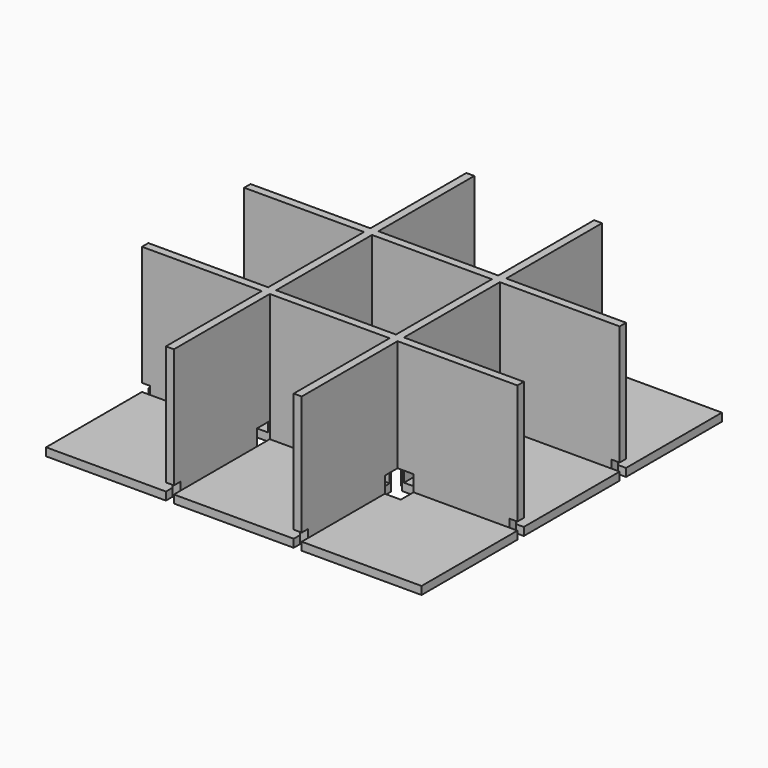
from build123d import *

# Parameters (mm, degrees)
F0_W     = 1
F0_H     = 15
F0_W_2   = 15
F0_H_2   = 1
F1_DEPTH = 1
F2_DEPTH = 16
F3_W     = 2
F3_H     = 3
F3_W_2   = 3
F3_H_2   = 2
F4_DEPTH = 3
F5_W     = 1
F5_H     = 1
F6_DEPTH = 25
F7_DEPTH = 15
F9_DEPTH = 1


with BuildPart() as f1:
    # F0 (on Top) → F1 (new body)
    with BuildSketch(Plane.XY):
        with Locations((8, 0)):
            Rectangle(F0_W, F0_H)
        with Locations((-16, -8)):
            Rectangle(F0_W_2, F0_H_2)
        with Locations((-16, 0)):
            Rectangle(F0_W_2, F0_H)
        with Locations((8, -16)):
            Rectangle(F0_W, F0_H)
        with Locations((0, -16)):
            Rectangle(F0_W_2, F0_H)
        with Locations((-8, -16)):
            Rectangle(F0_W, F0_H)
        with Locations((16, -16)):
            Rectangle(F0_W_2, F0_H)
        with Locations((-16, -16)):
            Rectangle(F0_W_2, F0_H)
        with Locations((16, 0)):
            Rectangle(F0_W_2, F0_H)
        with Locations((16, -8)):
            Rectangle(F0_W_2, F0_H_2)
        with Locations((0, -8)):
            Rectangle(F0_W_2, F0_H_2)
        with Locations((-8, 0)):
            Rectangle(F0_W, F0_H)
        Rectangle(F0_W_2, F0_H)
        with Locations((8, -8)):
            Rectangle(F0_W, F0_H_2)
        with Locations((-8, -8)):
            Rectangle(F0_W, F0_H_2)
        with Locations((-8, 8)):
            Rectangle(F0_W, F0_H_2)
        with Locations((-16, 8)):
            Rectangle(F0_W_2, F0_H_2)
        with Locations((8, 16)):
            Rectangle(F0_W, F0_H)
        with Locations((0, 16)):
            Rectangle(F0_W_2, F0_H)
        with Locations((-8, 16)):
            Rectangle(F0_W, F0_H)
        with Locations((16, 16)):
            Rectangle(F0_W_2, F0_H)
        with Locations((16, 8)):
            Rectangle(F0_W_2, F0_H_2)
        with Locations((-16, 16)):
            Rectangle(F0_W_2, F0_H)
        with Locations((8, 8)):
            Rectangle(F0_W, F0_H_2)
        with Locations((0, 8)):
            Rectangle(F0_W_2, F0_H_2)
    extrude(amount=-F1_DEPTH)

    # F0 (on Top) → F2 (join)
    with BuildSketch(Plane.XY):
        with Locations((-8, -8)):
            Rectangle(F0_W, F0_H_2)
        with Locations((8, -8)):
            Rectangle(F0_W, F0_H_2)
        with Locations((-8, 8)):
            Rectangle(F0_W, F0_H_2)
        with Locations((8, 8)):
            Rectangle(F0_W, F0_H_2)
        with Locations((16, 8)):
            Rectangle(F0_W_2, F0_H_2)
        with Locations((8, 16)):
            Rectangle(F0_W, F0_H)
        with Locations((-8, 16)):
            Rectangle(F0_W, F0_H)
        with Locations((0, 8)):
            Rectangle(F0_W_2, F0_H_2)
        with Locations((-16, 8)):
            Rectangle(F0_W_2, F0_H_2)
        with Locations((-8, 0)):
            Rectangle(F0_W, F0_H)
        with Locations((-16, -8)):
            Rectangle(F0_W_2, F0_H_2)
        with Locations((0, -8)):
            Rectangle(F0_W_2, F0_H_2)
        with Locations((16, -8)):
            Rectangle(F0_W_2, F0_H_2)
        with Locations((8, -16)):
            Rectangle(F0_W, F0_H)
        with Locations((-8, -16)):
            Rectangle(F0_W, F0_H)
        with Locations((8, 0)):
            Rectangle(F0_W, F0_H)
    extrude(amount=F2_DEPTH)

    # F3 (on face) → F4 (cut)
    with BuildSketch(Plane(origin=(0, 0, -1), x_dir=(1, 0, 0), z_dir=(0, 0, -1))):
        with BuildLine():
            Line((-7.5, 8.25), (-7.5, 7.5))
            Line((-7.5, 7.5), (-6.75, 7.5))
            ThreePointArc((-6.75, 7.5), (-6.9696699141, 8.0303300859), (-7.5, 8.25))
        make_face()
        with BuildLine():
            Line((-6.75, 7.5), (-7.5, 7.5))
            Line((-7.5, 7.5), (-7.5, 6.75))
            ThreePointArc((-7.5, 6.75), (-6.9696699141, 6.9696699141), (-6.75, 7.5))
        make_face()
        with BuildLine():
            Line((-7.5, 6.75), (-7.5, 7.5))
            Line((-7.5, 7.5), (-8.25, 7.5))
            ThreePointArc((-8.25, 7.5), (-8.0303300859, 6.9696699141), (-7.5, 6.75))
        make_face()
        with BuildLine():
            Line((-8.25, 7.5), (-7.5, 7.5))
            Line((-7.5, 7.5), (-7.5, 8.25))
            ThreePointArc((-7.5, 8.25), (-8.0303300859, 8.0303300859), (-8.25, 7.5))
        make_face()
        with BuildLine():
            Line((-1, 7.5), (-6.75, 7.5))
            ThreePointArc((-6.75, 7.5), (-6.9696699141, 6.9696699141), (-7.5, 6.75))
            Line((-7.5, 6.75), (-7.5, 1))
            Line((-7.5, 1), (-7.5, -1))
            Line((-7.5, -1), (-7.5, -6.75))
            ThreePointArc((-7.5, -6.75), (-6.9696699141, -6.9696699141), (-6.75, -7.5))
            Line((-6.75, -7.5), (-1, -7.5))
            Line((-1, -7.5), (1, -7.5))
            Line((1, -7.5), (6.75, -7.5))
            ThreePointArc((6.75, -7.5), (6.9696699141, -6.9696699141), (7.5, -6.75))
            Line((7.5, -6.75), (7.5, -1))
            Line((7.5, -1), (7.5, 1))
            Line((7.5, 1), (7.5, 6.75))
            ThreePointArc((7.5, 6.75), (6.9696699141, 6.9696699141), (6.75, 7.5))
            Line((6.75, 7.5), (1, 7.5))
            Line((1, 7.5), (-1, 7.5))
        make_face()
        with BuildLine():
            Line((-10.5, 7.5), (-8.25, 7.5))
            ThreePointArc((-8.25, 7.5), (-8.0303300859, 8.0303300859), (-7.5, 8.25))
            Line((-7.5, 8.25), (-7.5, 10.5))
            Line((-7.5, 10.5), (-10.5, 10.5))
            Line((-10.5, 10.5), (-10.5, 7.5))
        make_face()
        with Locations((0, 9)):
            Rectangle(F3_W, F3_H)
        with Locations((-9, 0)):
            Rectangle(F3_W_2, F3_H_2)
        with BuildLine():
            ThreePointArc((7.5, 8.25), (6.9696699141, 8.0303300859), (6.75, 7.5))
            Line((6.75, 7.5), (7.5, 7.5))
            Line((7.5, 7.5), (7.5, 8.25))
        make_face()
        with BuildLine():
            Line((7.5, 7.5), (6.75, 7.5))
            ThreePointArc((6.75, 7.5), (6.9696699141, 6.9696699141), (7.5, 6.75))
            Line((7.5, 6.75), (7.5, 7.5))
        make_face()
        with BuildLine():
            ThreePointArc((-6.75, -7.5), (-6.9696699141, -6.9696699141), (-7.5, -6.75))
            Line((-7.5, -6.75), (-7.5, -7.5))
            Line((-7.5, -7.5), (-6.75, -7.5))
        make_face()
        with BuildLine():
            Line((-7.5, -7.5), (-7.5, -6.75))
            ThreePointArc((-7.5, -6.75), (-8.0303300859, -6.9696699141), (-8.25, -7.5))
            Line((-8.25, -7.5), (-7.5, -7.5))
        make_face()
        with BuildLine():
            Line((8.25, 7.5), (7.5, 7.5))
            Line((7.5, 7.5), (7.5, 6.75))
            ThreePointArc((7.5, 6.75), (8.0303300859, 6.9696699141), (8.25, 7.5))
        make_face()
        with BuildLine():
            Line((7.5, 8.25), (7.5, 7.5))
            Line((7.5, 7.5), (8.25, 7.5))
            ThreePointArc((8.25, 7.5), (8.0303300859, 8.0303300859), (7.5, 8.25))
        make_face()
        with BuildLine():
            Line((7.5, 10.5), (7.5, 8.25))
            ThreePointArc((7.5, 8.25), (8.0303300859, 8.0303300859), (8.25, 7.5))
            Line((8.25, 7.5), (10.5, 7.5))
            Line((10.5, 7.5), (10.5, 10.5))
            Line((10.5, 10.5), (7.5, 10.5))
        make_face()
        with BuildLine():
            Line((-7.5, -8.25), (-7.5, -7.5))
            Line((-7.5, -7.5), (-8.25, -7.5))
            ThreePointArc((-8.25, -7.5), (-8.0303300859, -8.0303300859), (-7.5, -8.25))
        make_face()
        with BuildLine():
            Line((-6.75, -7.5), (-7.5, -7.5))
            Line((-7.5, -7.5), (-7.5, -8.25))
            ThreePointArc((-7.5, -8.25), (-6.9696699141, -8.0303300859), (-6.75, -7.5))
        make_face()
        with BuildLine():
            ThreePointArc((-7.5, -8.25), (-8.0303300859, -8.0303300859), (-8.25, -7.5))
            Line((-8.25, -7.5), (-10.5, -7.5))
            Line((-10.5, -7.5), (-10.5, -10.5))
            Line((-10.5, -10.5), (-7.5, -10.5))
            Line((-7.5, -10.5), (-7.5, -8.25))
        make_face()
        with Locations((9, 0)):
            Rectangle(F3_W_2, F3_H_2)
        with Locations((0, -9)):
            Rectangle(F3_W, F3_H)
        with BuildLine():
            ThreePointArc((8.25, -7.5), (8.0303300859, -6.9696699141), (7.5, -6.75))
            Line((7.5, -6.75), (7.5, -7.5))
            Line((7.5, -7.5), (8.25, -7.5))
        make_face()
        with BuildLine():
            Line((7.5, -7.5), (7.5, -6.75))
            ThreePointArc((7.5, -6.75), (6.9696699141, -6.9696699141), (6.75, -7.5))
            Line((6.75, -7.5), (7.5, -7.5))
        make_face()
        with BuildLine():
            Line((7.5, -7.5), (6.75, -7.5))
            ThreePointArc((6.75, -7.5), (6.9696699141, -8.0303300859), (7.5, -8.25))
            Line((7.5, -8.25), (7.5, -7.5))
        make_face()
        with BuildLine():
            Line((8.25, -7.5), (7.5, -7.5))
            Line((7.5, -7.5), (7.5, -8.25))
            ThreePointArc((7.5, -8.25), (8.0303300859, -8.0303300859), (8.25, -7.5))
        make_face()
        with BuildLine():
            Line((10.5, -7.5), (8.25, -7.5))
            ThreePointArc((8.25, -7.5), (8.0303300859, -8.0303300859), (7.5, -8.25))
            Line((7.5, -8.25), (7.5, -10.5))
            Line((7.5, -10.5), (10.5, -10.5))
            Line((10.5, -10.5), (10.5, -7.5))
        make_face()
    extrude(amount=-F4_DEPTH, mode=Mode.SUBTRACT)

    # F5 (on face) → F6 (cut)
    with BuildSketch(Plane.XY.offset(16)):
        with Locations((-8, 23)):
            Rectangle(F5_W, F5_H)
        with Locations((-23, 8)):
            Rectangle(F5_W, F5_H)
        with Locations((8, 23)):
            Rectangle(F5_W, F5_H)
        with Locations((23, 8)):
            Rectangle(F5_W, F5_H)
        with Locations((23, -8)):
            Rectangle(F5_W, F5_H)
        with Locations((8, -23)):
            Rectangle(F5_W, F5_H)
        with Locations((-8, -23)):
            Rectangle(F5_W, F5_H)
        with Locations((-23, -8)):
            Rectangle(F5_W, F5_H)
    extrude(amount=-F6_DEPTH, mode=Mode.SUBTRACT)

    # F5 (on face) → F7 (join)
    with BuildSketch(Plane.XY.offset(16)):
        with Locations((-8, 23)):
            Rectangle(F5_W, F5_H)
        with Locations((-23, 8)):
            Rectangle(F5_W, F5_H)
        with Locations((8, 23)):
            Rectangle(F5_W, F5_H)
        with Locations((23, 8)):
            Rectangle(F5_W, F5_H)
        with Locations((23, -8)):
            Rectangle(F5_W, F5_H)
        with Locations((8, -23)):
            Rectangle(F5_W, F5_H)
        with Locations((-8, -23)):
            Rectangle(F5_W, F5_H)
        with Locations((-23, -8)):
            Rectangle(F5_W, F5_H)
    extrude(amount=-F7_DEPTH)

    # F8 (on Top) → F9 (join)
    with BuildSketch(Plane.XY):
        Polygon((-1, 7.5), (-5.5, 7.5), (-5.5, 5.5), (-7.5, 5.5), (-7.5, 1), (-6.5, 1), (-6.5, -1), (-7.5, -1), (-7.5, -5.5), (-5.5, -5.5), (-5.5, -7.5), (-1, -7.5), (-1, -5.5), (1, -5.5), (1, -7.5), (5.5, -7.5), (5.5, -5.5), (7.5, -5.5), (7.5, -1), (5.5, -1), (5.5, 1), (7.5, 1), (7.5, 5.5), (5.5, 5.5), (5.5, 7.5), (1, 7.5), (1, 5.5), (-1, 5.5), align=None)
    extrude(amount=F9_DEPTH)


solid = f1.part
